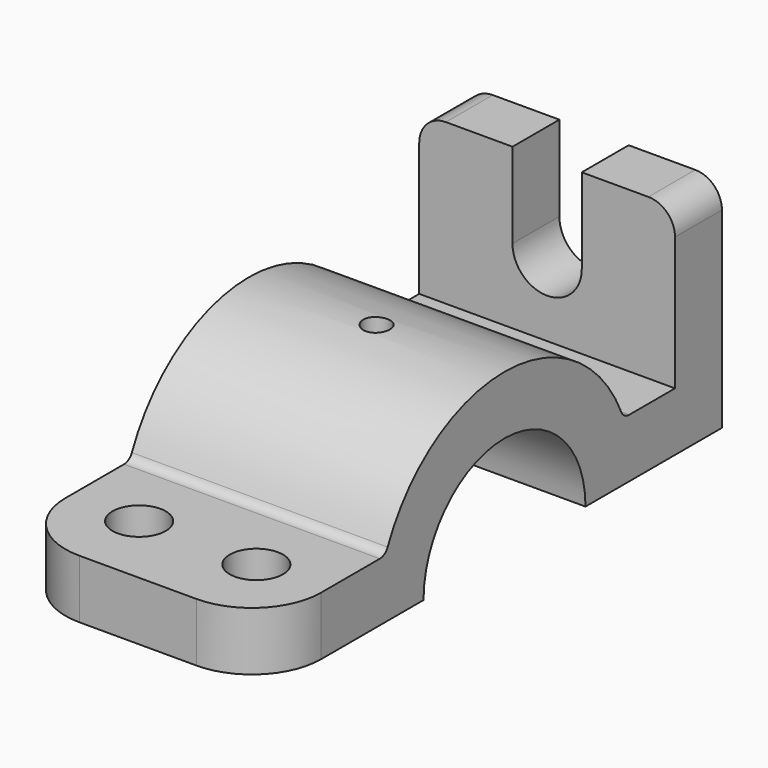
from build123d import *

# Parameters (mm, degrees)
F0_W     = 11
F0_H     = 30
F1_DEPTH = 24
F3_DEPTH = 11
F4_R     = 2.5
F4_R_2   = 5
F5_DEPTH = 41.001
F6_R     = 13
F7_R     = 5
F8_R     = 2


with BuildPart() as f1:
    # F0 (on Right) → F1 (new body, symmetric)
    with BuildSketch(Plane.YZ):
        with BuildLine():
            ThreePointArc((15.4919333848, 11), (18.1017503893, 5.7729223833), (19, 0))
            Line((19, 0), (30, 0))
            ThreePointArc((30, 0), (29.4730143031, 5.5983415304), (27.9105714739, 11))
            Line((27.9105714739, 11), (15.4919333848, 11))
        make_face()
        with BuildLine():
            ThreePointArc((-15.4919333848, 11), (0, 19), (15.4919333848, 11))
            Line((15.4919333848, 11), (27.9105714739, 11))
            ThreePointArc((27.9105714739, 11), (0, 30), (-27.9105714739, 11))
            Line((-27.9105714739, 11), (-15.4919333848, 11))
        make_face()
        with BuildLine():
            Line((-30, 0), (-19, 0))
            ThreePointArc((-19, 0), (-18.1017503893, 5.7729223833), (-15.4919333848, 11))
            Line((-15.4919333848, 11), (-27.9105714739, 11))
            ThreePointArc((-27.9105714739, 11), (-29.4730143031, 5.5983415304), (-30, 0))
        make_face()
        with BuildLine():
            ThreePointArc((27.9105714739, 11), (29.4730143031, 5.5983415304), (30, 0))
            Line((30, 0), (51, 0))
            Line((51, 0), (51, 11))
            Line((51, 11), (40, 11))
            Line((40, 11), (27.9105714739, 11))
        make_face()
        with BuildLine():
            Line((-56, 0), (-30, 0))
            ThreePointArc((-30, 0), (-29.4730143031, 5.5983415304), (-27.9105714739, 11))
            Line((-27.9105714739, 11), (-56, 11))
            Line((-56, 11), (-56, 0))
        make_face()
        with Locations((45.5, 26)):
            Rectangle(F0_W, F0_H)
    extrude(amount=F1_DEPTH, both=True)

    # F2 (on face) → F3 (cut, through all)
    with BuildSketch(Plane(origin=(0, 51, 0), x_dir=(-1, 0, 0), z_dir=(0, 1, 0))):
        with BuildLine():
            ThreePointArc((-6.5, 25), (0, 18.5), (6.5, 25))
            ThreePointArc((6.5, 25), (0, 31.5), (-6.5, 25))
        make_face()
        with BuildLine():
            ThreePointArc((-6.5, 25), (0, 31.5), (6.5, 25))
            Line((6.5, 25), (6.5, 41))
            Line((6.5, 41), (-6.5, 41))
            Line((-6.5, 41), (-6.5, 25))
        make_face()
    extrude(amount=-F3_DEPTH, mode=Mode.SUBTRACT)

    # F4 (on Top) → F5 (cut, through all)
    with BuildSketch(Plane.XY):
        Circle(F4_R)
        with Locations((-11, -41.955285737)):
            Circle(F4_R_2)
        with Locations((11, -41.955285737)):
            Circle(F4_R_2)
    extrude(amount=F5_DEPTH, mode=Mode.SUBTRACT)

    # F6
    f6_edges = [f1.edges().sort_by_distance(p)[0] for p in [
        (24, -56, 5.5),
        (-24, -56, 5.5),
    ]]
    fillet(f6_edges, radius=F6_R)

    # F7
    f7_edges = [f1.edges().sort_by_distance(p)[0] for p in [
        (24, 45.5, 41),
        (-24, 45.5, 41),
    ]]
    fillet(f7_edges, radius=F7_R)

    # F8
    f8_edges = [f1.edges().sort_by_distance(p)[0] for p in [
        (0, -27.910571, 11),
        (0, 27.910571, 11),
    ]]
    fillet(f8_edges, radius=F8_R)


solid = f1.part
